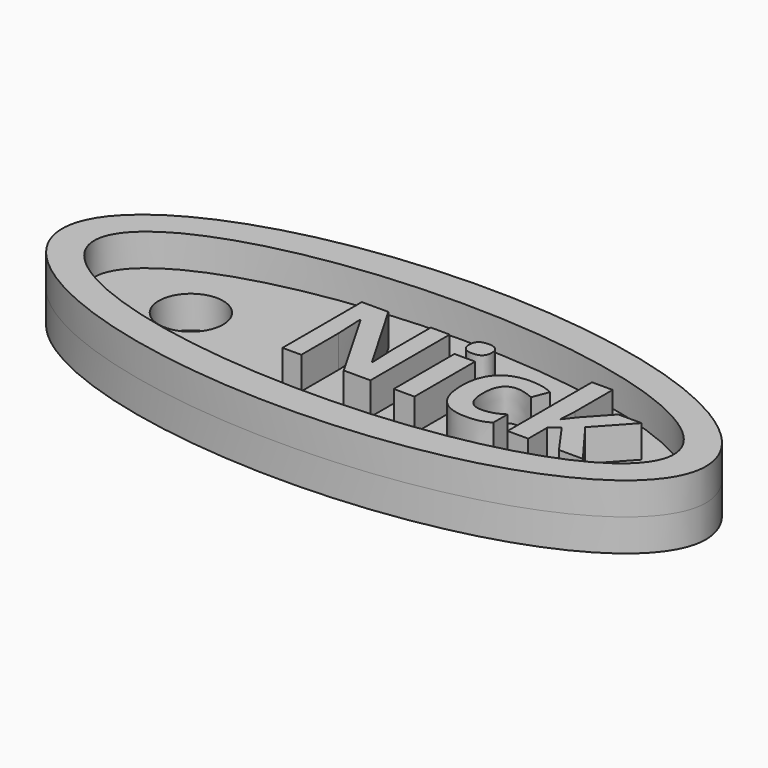
from build123d import *

# Parameters (mm, degrees)
F1_DEPTH     = 3.175
F3_DEPTH     = 3.175
F4_TEXT_SIZE = 13.7001538547
F5_DEPTH     = 3.175
F6_R         = 3.175
F7_DEPTH     = 3.1760001


# Not quite as in the source:
# - Text() gives the source's letters only with a copy of the font that has no kerning and outlines rounded to 1/6400 em; it was checked with that copy


with BuildPart() as f1:
    # F0 (on Top) → F1 (new body, symmetric)
    with BuildSketch(Plane.XY):
        with BuildLine():
            add(Edge.make_bspline(
                [(31.75, 0), (31.75, 21.9970452561), (-15.875, 10.9985226281), (-63.5, 0), (-15.875, -10.9985226281), (31.75, -21.9970452561), (31.75, 0)],
                knots=[0, 0, 0, 2.0943951024, 2.0943951024, 4.1887902048, 4.1887902048, 6.2831853072, 6.2831853072, 6.2831853072], degree=2, weights=[1, 0.5, 1, 0.5, 1, 0.5, 1]))
        make_face()
    extrude(amount=F1_DEPTH, both=True)

    # F2 (on face) → F3 (cut)
    with BuildSketch(Plane.XY.offset(3.175)):
        with BuildLine():
            add(Edge.make_bspline(
                [(28.575, 0), (28.575, 16.4977839421), (-14.2875, 8.248891971), (-57.15, 0), (-14.2875, -8.248891971), (28.575, -16.4977839421), (28.575, 0)],
                knots=[0, 0, 0, 2.0943951024, 2.0943951024, 4.1887902048, 4.1887902048, 6.2831853072, 6.2831853072, 6.2831853072], degree=2, weights=[1, 0.5, 1, 0.5, 1, 0.5, 1]))
        make_face()
    extrude(amount=-F3_DEPTH, mode=Mode.SUBTRACT)

    # F4 (on face) → F5 (join)
    with BuildSketch(Plane.XY):
        with Locations((-7.3020236718, -4.9320553877)):
            Text('Nick', F4_TEXT_SIZE, font='Open Sans', font_style=FontStyle.BOLD, text_align=(TextAlign.LEFT, TextAlign.BOTTOM))
    extrude(amount=F5_DEPTH)

    # F6 (on face) → F7 (cut, through all)
    with BuildSketch(Plane.XY):
        with Locations((-19.05, 0)):
            Circle(F6_R)
    extrude(amount=-F7_DEPTH, mode=Mode.SUBTRACT)


solid = f1.part
